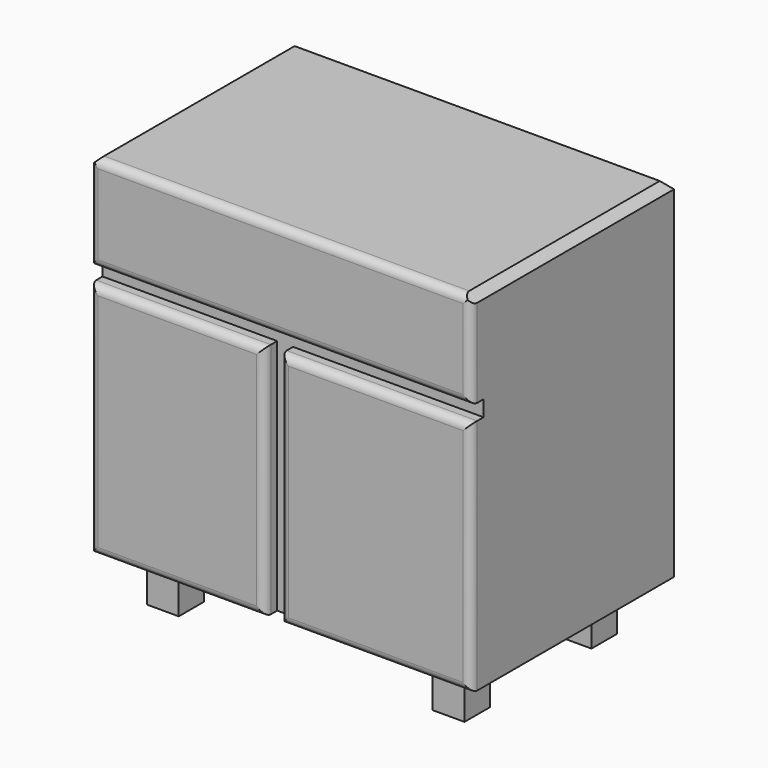
from build123d import *

# Parameters (mm, degrees)
F0_W         = 609.6
F0_H         = 381
F1_DEPTH     = 635
F2_DEPTH     = 25.4
F3_W         = 50.8
F3_H         = 76.2
F3_W_2       = 406.4
F4_DEPTH     = 1574.8
F5_W         = 50.8
F5_H         = 76.2
F5_W_2       = 203.2
F6_DEPTH     = 970.28
F7_W         = 25.4
F7_H         = 379.8168087482
F8_DEPTH     = 25.4
F9_R         = 12.7
F10_T1_DEPTH = 459.0207478943
F10_T3_DEPTH = 674.9207478943


# Not quite as in the source:
# - a fillet or chamfer that OpenCascade refuses, or shapes differently, is made with other operations: its cross-section is extruded or revolved along the edge and cut away or added


with BuildPart() as f1:
    # F0 (on Top) → F1 (new body)
    with BuildSketch(Plane.XY):
        with Locations((304.8, 190.5)):
            Rectangle(F0_W, F0_H)
    extrude(amount=F1_DEPTH)

    # F2 (add): a face of the model
    f2_faces = [f1.faces().sort_by_distance(p)[0] for p in [
        (304.8, 0, 317.5),
    ]]
    extrude(f2_faces, amount=F2_DEPTH)

    # F3 (on face) → F4 (cut)
    with BuildSketch(Plane.XZ.offset(25.4)):
        with Locations((25.4, 38.1)):
            Rectangle(F3_W, F3_H)
        with Locations((304.8, 38.1)):
            Rectangle(F3_W_2, F3_H)
        with Locations((584.2, 38.1)):
            Rectangle(F3_W, F3_H)
    extrude(amount=-F4_DEPTH, mode=Mode.SUBTRACT)

    # F5 (on face) → F6 (cut)
    with BuildSketch(Plane.YZ.offset(558.8)):
        with Locations((0, 38.1)):
            Rectangle(F5_W, F5_H)
        with Locations((177.8, 38.1)):
            Rectangle(F5_W_2, F5_H)
        with Locations((355.6, 38.1)):
            Rectangle(F5_W, F5_H)
    extrude(amount=-F6_DEPTH, mode=Mode.SUBTRACT)

    # F7 (on face) → F8 (cut)
    with BuildSketch(Plane.XZ.offset(25.4)):
        with Locations((292.1, 266.1084043741)):
            Rectangle(F7_W, F7_H)
        Polygon((609.6, 481.4168087482), (0, 481.4168087482), (0, 456.0168087482), (279.4, 456.0168087482), (304.8, 456.0168087482), (609.6, 456.0168087482), align=None)
    extrude(amount=-F8_DEPTH, mode=Mode.SUBTRACT)

    # F9
    f9_edges = [f1.edges().sort_by_distance(p)[0] for p in [
        (609.6, -25.4, 558.208404),
        (304.8, -25.4, 635),
        (0, -25.4, 558.208404),
        (304.8, -25.4, 481.416809),
        (279.4, -25.4, 266.108404),
        (139.7, -25.4, 456.016809),
        (0, -25.4, 266.108404),
        (139.7, -25.4, 76.2),
        (609.6, -25.4, 266.108404),
        (457.2, -25.4, 456.016809),
        (304.8, -25.4, 266.108404),
        (457.2, -25.4, 76.2),
    ]]
    fillet(f9_edges, radius=F9_R)

    # F10: chamfer of 12.7 on 4 edges, made by hand

    # F10_s2 → F10_t1 (cut)
    with BuildSketch(Plane.XZ.offset(-413.6603739472)):
        Polygon((0, 622.3), (12.7, 635), (0, 635), align=None)
        Polygon((596.9, 635), (609.6, 622.3), (609.6, 635), align=None)
    extrude(amount=F10_T1_DEPTH, mode=Mode.SUBTRACT)

    # F10_s4 → F10_t3 (cut)
    with BuildSketch(Plane.YZ.offset(-32.6603739472)):
        Polygon((381, 622.3), (368.3, 635), (381, 635), align=None)
    extrude(amount=F10_T3_DEPTH, mode=Mode.SUBTRACT)


solid = f1.part
